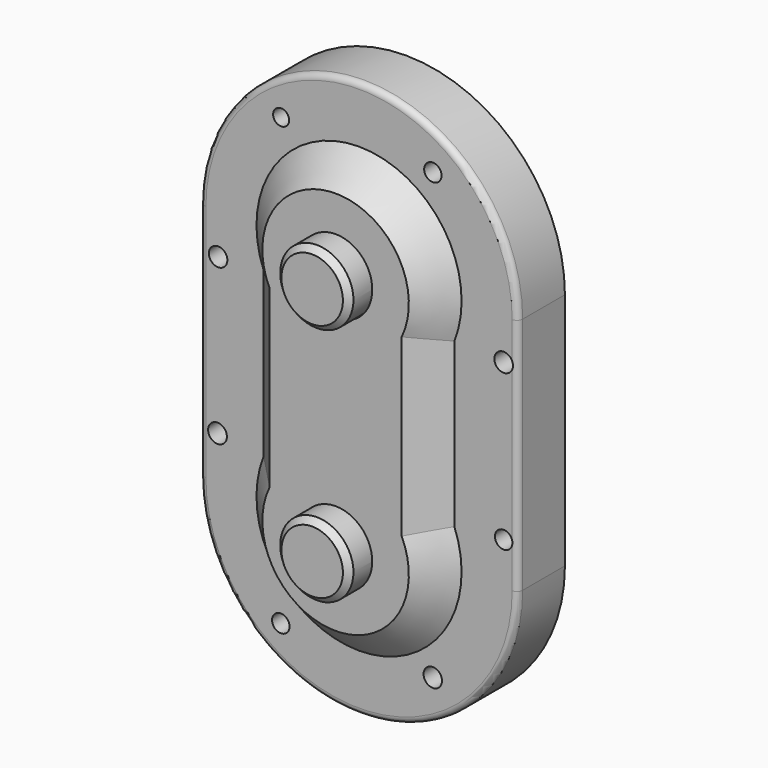
from build123d import *

# Parameters (mm, degrees)
F0_R        = 7.5832559133
F0_R_2      = 8.1429677051
F0_R_3      = 7.9975424125
F0_R_4      = 7.5832754374
F0_R_5      = 8.0140482533
F0_R_6      = 6.9266770474
F0_R_7      = 8.0650025084
F0_R_8      = 7.5399035307
F1_DEPTH    = 50.8
F0_R_9      = 38.1
F0_R_10     = 31.75
F2_DEPTH    = 25.4
F4_R        = 31.75
F5_DEPTH    = 38.1
F6_SIZE     = 5.08
F7_T1_DEPTH = 206.9338
F7_T4_ANGLE = 180
F7_T6_ANGLE = 180
F8_SIZE     = 25.39999


# Not quite as in the source:
# - a fillet or chamfer that OpenCascade refuses, or shapes differently, is made with other operations: its cross-section is extruded or revolved along the edge and cut away or added
# - a fillet or chamfer is up to 0.001 mm smaller than in the source, because OpenCascade refuses the exact size


with BuildPart() as f1:
    # F0 (on Front) → F1 (new body)
    with BuildSketch(Plane.XZ):
        with BuildLine():
            Line((137.8331, -103.4669), (137.8331, 103.4669))
            ThreePointArc((137.8331, 103.4669), (0, 241.3), (-137.8331, 103.4669))
            Line((-137.8331, 103.4669), (-137.8331, -103.4669))
            ThreePointArc((-137.8331, -103.4669), (0, -241.3), (137.8331, -103.4669))
        make_face()
        with Locations((-67.8210385144, -193.5505885762)):
            Circle(F0_R, mode=Mode.SUBTRACT)
        with Locations((-122.6988486946, -66.3264859599)):
            Circle(F0_R_2, mode=Mode.SUBTRACT)
        with Locations((63.9354459941, -192.0185405892)):
            Circle(F0_R_3, mode=Mode.SUBTRACT)
        with Locations((125.382462889, -66.8681580704)):
            Circle(F0_R_4, mode=Mode.SUBTRACT)
        with Locations((-122.1571840346, 68.5286801177)):
            Circle(F0_R_5, mode=Mode.SUBTRACT)
        with Locations((-67.5374619663, 192.7409227806)):
            Circle(F0_R_6, mode=Mode.SUBTRACT)
        with BuildLine():
            ThreePointArc((-82.6771222469, 70.7911680728), (0, 192.3669), (82.6771222469, 70.7911680728))
            Line((82.6771222469, 70.7911680728), (82.6771222469, -70.7911680728))
            ThreePointArc((82.6771222469, -70.7911680728), (0, -192.3669), (-82.6771222469, -70.7911680728))
            Line((-82.6771222469, -70.7911680728), (-82.6771222469, 70.7911680728))
        make_face(mode=Mode.SUBTRACT)
        with Locations((125.382462889, 68.5286801177)):
            Circle(F0_R_7, mode=Mode.SUBTRACT)
        with Locations((63.9896340668, 193.4904660898)):
            Circle(F0_R_8, mode=Mode.SUBTRACT)
    extrude(amount=-F1_DEPTH)

    # F7: fillet of radius 5.08 on 4 edges, made by hand

    # F7_s2 → F7_t1 (cut)
    with BuildSketch(Plane.XY.offset(-103.4669)):
        with BuildLine():
            ThreePointArc((137.8331, 5.08), (136.3452024484, 1.4878975516), (132.7531, 0))
            Line((132.7531, 0), (137.8331, 0))
            Line((137.8331, 0), (137.8331, 5.08))
        make_face()
        with BuildLine():
            ThreePointArc((-137.8331, 5.08), (-136.3452024484, 1.4878975516), (-132.7531, 0))
            Line((-132.7531, 0), (-137.8331, 0))
            Line((-137.8331, 0), (-137.8331, 5.08))
        make_face()
    extrude(amount=F7_T1_DEPTH, mode=Mode.SUBTRACT)

    # F7_s3 → F7_t4 (revolve, cut)
    with BuildSketch(Plane.XY.offset(103.4669)):
        with BuildLine():
            ThreePointArc((137.8331, 5.08), (136.3452024484, 1.4878975516), (132.7531, 0))
            Line((132.7531, 0), (137.8331, 0))
            Line((137.8331, 0), (137.8331, 5.08))
        make_face()
    revolve(axis=Axis((0, 0, 103.4669), (0, -1, 0)), revolution_arc=F7_T4_ANGLE, mode=Mode.SUBTRACT)

    # F7_s5 → F7_t6 (revolve, cut)
    with BuildSketch(Plane.XY.offset(-103.4669)):
        with BuildLine():
            ThreePointArc((-137.8331, 5.08), (-136.3452024484, 1.4878975516), (-132.7531, 0))
            Line((-132.7531, 0), (-137.8331, 0))
            Line((-137.8331, 0), (-137.8331, 5.08))
        make_face()
    revolve(axis=Axis((0, 0, -103.4669), (0, -1, 0)), revolution_arc=F7_T6_ANGLE, mode=Mode.SUBTRACT)


with BuildPart() as f2:
    # F0 (on Front) → F2 (new body)
    with BuildSketch(Plane.XZ):
        with BuildLine():
            Line((82.6771222469, -70.7911680728), (82.6771222469, 70.7911680728))
            ThreePointArc((82.6771222469, 70.7911680728), (0, 192.3669), (-82.6771222469, 70.7911680728))
            Line((-82.6771222469, 70.7911680728), (-82.6771222469, -70.7911680728))
            ThreePointArc((-82.6771222469, -70.7911680728), (0, -192.3669), (82.6771222469, -70.7911680728))
        make_face()
        with Locations((0, -103.4669)):
            Circle(F0_R_9, mode=Mode.SUBTRACT)
        with Locations((0, 103.4669)):
            Circle(F0_R_9, mode=Mode.SUBTRACT)
        with Locations((0, 103.4669)):
            Circle(F0_R_9)
        with Locations((0, 103.4669)):
            Circle(F0_R_10, mode=Mode.SUBTRACT)
        with Locations((0, -103.4669)):
            Circle(F0_R_9)
        with Locations((0, -103.4669)):
            Circle(F0_R_10, mode=Mode.SUBTRACT)
    extrude(amount=F2_DEPTH)

    # F4 (on offset) → F5 (join)
    with BuildSketch(Plane.XZ.offset(50.8)):
        with Locations((0, 104.1518346508)):
            Circle(F4_R)
        with Locations((0, -103.5747896099)):
            Circle(F4_R)
    extrude(amount=-F5_DEPTH)

    # F6
    f6_edges = [f2.edges().sort_by_distance(p)[0] for p in [
        (-31.75, -50.8, 104.151835),
        (-31.75, -50.8, -103.57479),
    ]]
    chamfer(f6_edges, length=F6_SIZE)

    # F8 (size 25.4 in the source; OpenCascade refuses exactly that, so slightly less here)
    f8_edges = [f2.edges().sort_by_distance(p)[0] for p in [
        (0, -25.4, 192.3669),
        (82.677122, -25.4, 0),
        (-82.677122, -25.4, 0),
        (0, -25.4, -192.3669),
    ]]
    chamfer(f8_edges, length=F8_SIZE)


solid = Compound([f1.part, f2.part])
